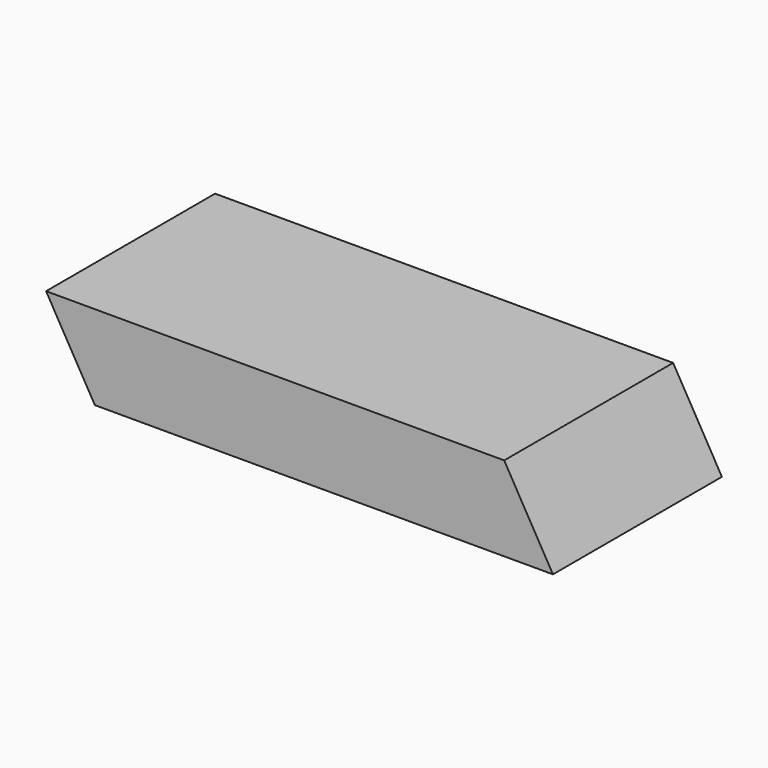
from build123d import *

# Parameters (mm, degrees)
F0_W     = 152.4
F0_H     = 63.5
F1_DEPTH = 25.4
F2_SIZE2 = 14.664687
F2_SIZE  = 25.39999
F3_SIZE2 = 14.664687
F3_SIZE  = 25.39999


# Not quite as in the source:
# - a fillet or chamfer is up to 0.001 mm smaller than in the source, because OpenCascade refuses the exact size


with BuildPart() as f1:
    # F0 (on Top) → F1 (new body)
    with BuildSketch(Plane.XY):
        with Locations((8.8605511625, -31.75)):
            Rectangle(F0_W, F0_H)
    extrude(amount=F1_DEPTH)

    # F2 (size 25.4 and 14.6646968374 in the source; OpenCascade refuses exactly that, so slightly less here)
    f2_edges = [f1.edges().sort_by_distance(p)[0] for p in [
        (85.060551, -31.75, 25.4),
    ]]
    f2_side = f1.faces().sort_by_distance((85.060551, -31.75, 12.7))[0]
    chamfer(f2_edges, length=F2_SIZE, length2=F2_SIZE2, reference=f2_side)

    # F3 (size 25.4 and 14.6646968374 in the source; OpenCascade refuses exactly that, so slightly less here)
    f3_edges = [f1.edges().sort_by_distance(p)[0] for p in [
        (-67.339449, -31.75, 0),
    ]]
    f3_side = f1.faces().sort_by_distance((-67.339449, -31.75, 12.7))[0]
    chamfer(f3_edges, length=F3_SIZE, length2=F3_SIZE2, reference=f3_side)


solid = f1.part
